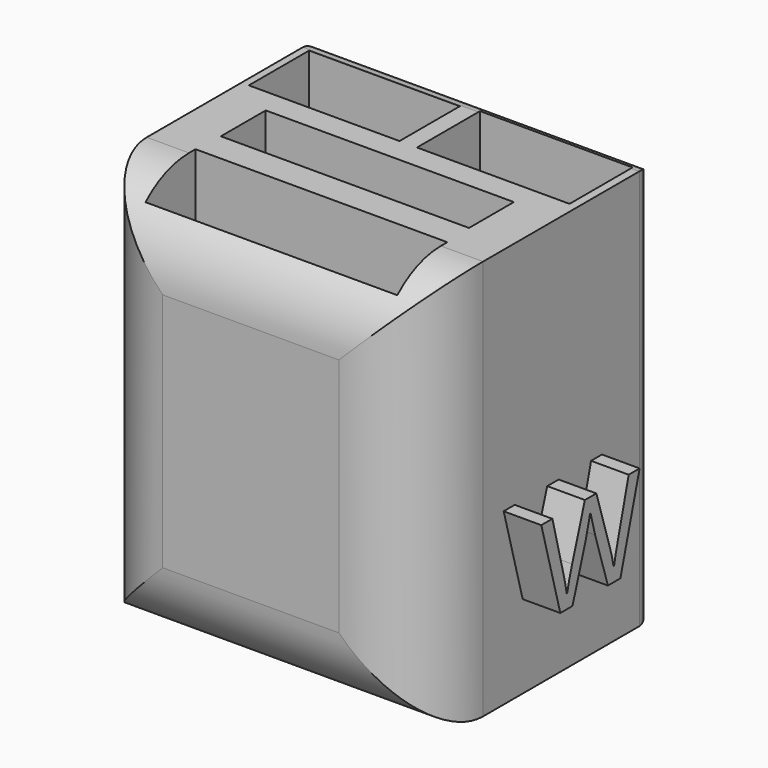
from build123d import *

# Parameters (mm, degrees)
F0_W         = 106.6799983382
F0_H         = 92.3977121711
F1_DEPTH     = 127
F2_W         = 47.801963985
F2_H         = 23.9009857178
F2_W_2       = 48.3849197626
F2_H_2       = 25.0668860972
F2_W_3       = 78.6983594298
F2_H_3       = 17.7800003439
F2_W_4       = 79.8642635345
F2_H_4       = 19.8203288019
F3_DEPTH     = 88.9
F4_T1_DEPTH  = 254
F4_T3_DEPTH  = 233.6799983382
F5_T1_DEPTH  = 152.4
F5_T3_DEPTH  = 132.0799983382
F6_TEXT_SIZE = 51.5672401836
F7_DEPTH     = 11.938


# Not quite as in the source:
# - a fillet or chamfer that OpenCascade refuses, or shapes differently, is made with other operations: its cross-section is extruded or revolved along the edge and cut away or added
# - Text() gives the source's letters only with a copy of the font that has no kerning and outlines rounded to 1/6400 em; it was checked with that copy


with BuildPart() as f1:
    # F0 (on Top) → F1 (new body)
    with BuildSketch(Plane.XY):
        Rectangle(F0_W, F0_H)
    extrude(amount=F1_DEPTH)

    # F2 (on face) → F3 (cut)
    with BuildSketch(Plane.XY.offset(127)):
        with Locations((-27.1072126925, 28.7103280425)):
            Rectangle(F2_W, F2_H)
        with Locations((26.5242606401, 29.2932782322)):
            Rectangle(F2_W_2, F2_H_2)
        Rectangle(F2_W_3, F2_H_3)
        with Locations((0, -28.1273778528)):
            Rectangle(F2_W_4, F2_H_4)
    extrude(amount=-F3_DEPTH, mode=Mode.SUBTRACT)

    # F4: fillet of radius 25.4 on 4 edges, made by hand

    # F4_s2 → F4_t1 (cut)
    with BuildSketch(Plane.XY.offset(-63.5)):
        with BuildLine():
            ThreePointArc((-27.9399991691, -46.1988560855), (-45.9005114112, -38.7593683277), (-53.3399991691, -20.7988560855))
            Line((-53.3399991691, -20.7988560855), (-53.3399991691, -46.1988560855))
            Line((-53.3399991691, -46.1988560855), (-27.9399991691, -46.1988560855))
        make_face()
        with BuildLine():
            ThreePointArc((27.9399991691, -46.1988560855), (45.9005114112, -38.7593683277), (53.3399991691, -20.7988560855))
            Line((53.3399991691, -20.7988560855), (53.3399991691, -46.1988560855))
            Line((53.3399991691, -46.1988560855), (27.9399991691, -46.1988560855))
        make_face()
    extrude(amount=F4_T1_DEPTH, mode=Mode.SUBTRACT)

    # F4_s4 → F4_t3 (cut)
    with BuildSketch(Plane.YZ.offset(-116.8399991691)):
        with BuildLine():
            ThreePointArc((-46.1988560855, 25.4), (-38.7593683277, 7.4394877579), (-20.7988560855, 0))
            Line((-20.7988560855, 0), (-46.1988560855, 0))
            Line((-46.1988560855, 0), (-46.1988560855, 25.4))
        make_face()
        with BuildLine():
            ThreePointArc((-46.1988560855, 101.6), (-38.7593683277, 119.5605122421), (-20.7988560855, 127))
            Line((-20.7988560855, 127), (-46.1988560855, 127))
            Line((-46.1988560855, 127), (-46.1988560855, 101.6))
        make_face()
    extrude(amount=F4_T3_DEPTH, mode=Mode.SUBTRACT)

    # F5: fillet of radius 5.08 on 4 edges, made by hand

    # F5_s2 → F5_t1 (cut)
    with BuildSketch(Plane.XY.offset(-12.7)):
        with BuildLine():
            ThreePointArc((53.3399991691, 41.1188560855), (51.8521016175, 44.710958534), (48.2599991691, 46.1988560855))
            Line((48.2599991691, 46.1988560855), (53.3399991691, 46.1988560855))
            Line((53.3399991691, 46.1988560855), (53.3399991691, 41.1188560855))
        make_face()
        with BuildLine():
            ThreePointArc((-53.3399991691, 41.1188560855), (-51.8521016175, 44.710958534), (-48.2599991691, 46.1988560855))
            Line((-48.2599991691, 46.1988560855), (-53.3399991691, 46.1988560855))
            Line((-53.3399991691, 46.1988560855), (-53.3399991691, 41.1188560855))
        make_face()
    extrude(amount=F5_T1_DEPTH, mode=Mode.SUBTRACT)

    # F5_s4 → F5_t3 (cut)
    with BuildSketch(Plane.YZ.offset(-66.0399991691)):
        with BuildLine():
            ThreePointArc((41.1188560855, 0), (44.710958534, 1.4878975516), (46.1988560855, 5.08))
            Line((46.1988560855, 5.08), (46.1988560855, 0))
            Line((46.1988560855, 0), (41.1188560855, 0))
        make_face()
        with BuildLine():
            ThreePointArc((41.1188560855, 127), (44.710958534, 125.5121024484), (46.1988560855, 121.92))
            Line((46.1988560855, 121.92), (46.1988560855, 127))
            Line((46.1988560855, 127), (41.1188560855, 127))
        make_face()
    extrude(amount=F5_T3_DEPTH, mode=Mode.SUBTRACT)

    # F6 (on face) → F7 (join)
    with BuildSketch(Plane.YZ.offset(53.3399991691)):
        with Locations((-13.2135516033, 26.3715870678)):
            Text('w', F6_TEXT_SIZE, font='Open Sans', text_align=(TextAlign.LEFT, TextAlign.BOTTOM))
    extrude(amount=F7_DEPTH)


solid = f1.part
